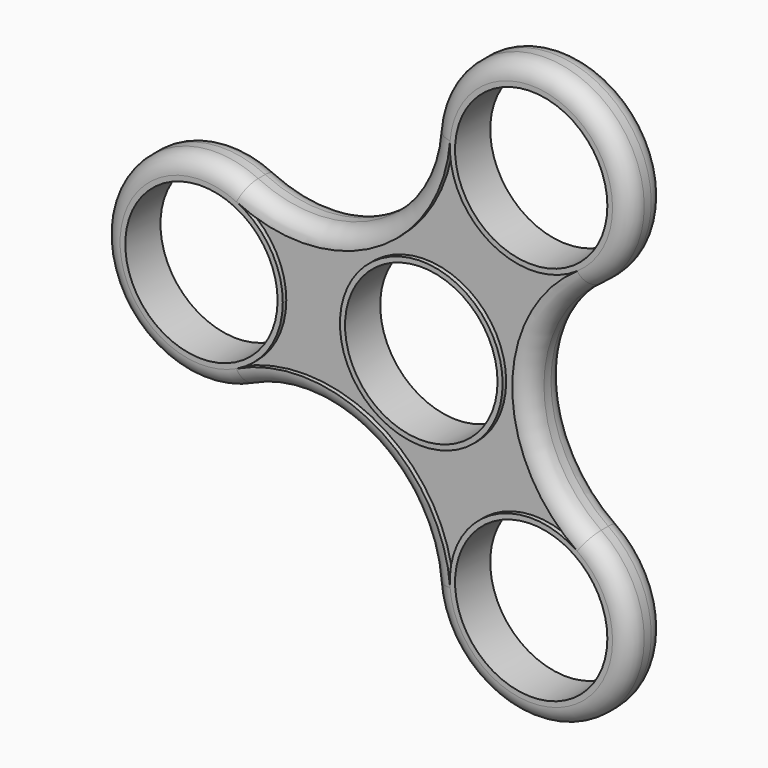
from build123d import *

# Parameters (mm, degrees)
F0_R     = 10.9982
F0_R_2   = 14.2875
F1_DEPTH = 6.35
F2_R     = 14.2875
F2_R_2   = 11.0109
F3_DEPTH = 6.35
F4_R     = 2.54
F5_R     = 11.7475
F6_DEPTH = 0.635
F7_R     = 11.7475
F8_DEPTH = 0.635


# Not quite as in the source:
# - a feature names something its author has since deleted; it is built from what else it names


with BuildPart() as f1:
    # F0 (on Front) → F1 (new body)
    with BuildSketch(Plane.XZ):
        with BuildLine():
            ThreePointArc((23.9537934556, -15.7121751829), (15.6755180632, 0), (23.9537934556, 15.7121751829))
            ThreePointArc((23.9537934556, 15.7121751829), (23.01875, 39.8696445267), (1.6302461293, 28.6006812411))
            ThreePointArc((1.6302461293, 28.6006812411), (-7.8377590316, 13.5753968602), (-25.584039585, 12.8885060581))
            ThreePointArc((-25.584039585, 12.8885060581), (-46.0375, 0), (-25.584039585, -12.8885060581))
            ThreePointArc((-25.584039585, -12.8885060581), (-7.8377590316, -13.5753968602), (1.6302461293, -28.6006812411))
            ThreePointArc((1.6302461293, -28.6006812411), (23.01875, -39.8696445267), (23.9537934556, -15.7121751829))
        make_face()
        with Locations((15.875, -27.4963065702)):
            Circle(F0_R, mode=Mode.SUBTRACT)
        with Locations((-31.75, 0)):
            Circle(F0_R, mode=Mode.SUBTRACT)
        Circle(F0_R_2, mode=Mode.SUBTRACT)
        with Locations((15.875, 27.4963065702)):
            Circle(F0_R, mode=Mode.SUBTRACT)
    extrude(amount=F1_DEPTH)

    # F2 (on face) → F3 (join)
    with BuildSketch(Plane.XZ.offset(6.35)):
        Circle(F2_R)
        Circle(F2_R_2, mode=Mode.SUBTRACT)
    extrude(amount=-F3_DEPTH)

    # F4
    f4_edges = [f1.edges().sort_by_distance(p)[0] for p in [
        (-7.837759, -6.35, 13.575397),
        (15.675518, 0, 0),
    ]]
    fillet(f4_edges, radius=F4_R)

    # F5 (on face) → F6 (cut)
    with BuildSketch(Plane.XZ.offset(6.35)):
        with BuildLine():
            ThreePointArc((-20.0025, 0), (-21.8111592615, -6.2628428867), (-26.6802103254, -10.5972160922))
            ThreePointArc((-26.6802103254, -10.5972160922), (-6.5677590316, -11.3756923346), (4.1626468174, -28.4043479662))
            ThreePointArc((4.1626468174, -28.4043479662), (10.00125, -17.3226731392), (22.517563508, -17.807131874))
            ThreePointArc((22.517563508, -17.807131874), (13.1355180632, 0), (22.517563508, 17.807131874))
            ThreePointArc((22.517563508, 17.807131874), (10.00125, 17.3226731392), (4.1626468174, 28.4043479662))
            ThreePointArc((4.1626468174, 28.4043479662), (-6.5677590316, 11.3756923346), (-26.6802103254, 10.5972160922))
            ThreePointArc((-26.6802103254, 10.5972160922), (-21.8111592615, 6.2628428867), (-20.0025, 0))
        make_face()
        Circle(F5_R, mode=Mode.SUBTRACT)
    extrude(amount=-F6_DEPTH, mode=Mode.SUBTRACT)

    # F7 (on face) → F8 (cut)
    with BuildSketch(Plane(origin=(0, 0, 0), x_dir=(-1, 0, 0), z_dir=(0, 1, 0))):
        with BuildLine():
            ThreePointArc((-4.1275, -27.4963065702), (-4.1362899929, -27.9506672407), (-4.1626468174, -28.4043479662))
            ThreePointArc((-4.1626468174, -28.4043479662), (6.5677590316, -11.3756923346), (26.6802103254, -10.5972160922))
            ThreePointArc((26.6802103254, -10.5972160922), (20.0025, 0), (26.6802103254, 10.5972160922))
            ThreePointArc((26.6802103254, 10.5972160922), (6.5677590316, 11.3756923346), (-4.1626468174, 28.4043479662))
            ThreePointArc((-4.1626468174, 28.4043479662), (-4.1362899929, 27.9506672407), (-4.1275, 27.4963065702))
            ThreePointArc((-4.1275, 27.4963065702), (-10.3991328796, 17.1031051611), (-22.517563508, 17.807131874))
            ThreePointArc((-22.517563508, 17.807131874), (-13.1355180632, 0), (-22.517563508, -17.807131874))
            ThreePointArc((-22.517563508, -17.807131874), (-10.3991328796, -17.1031051611), (-4.1275, -27.4963065702))
        make_face()
        Circle(F7_R, mode=Mode.SUBTRACT)
    extrude(amount=-F8_DEPTH, mode=Mode.SUBTRACT)


solid = f1.part
